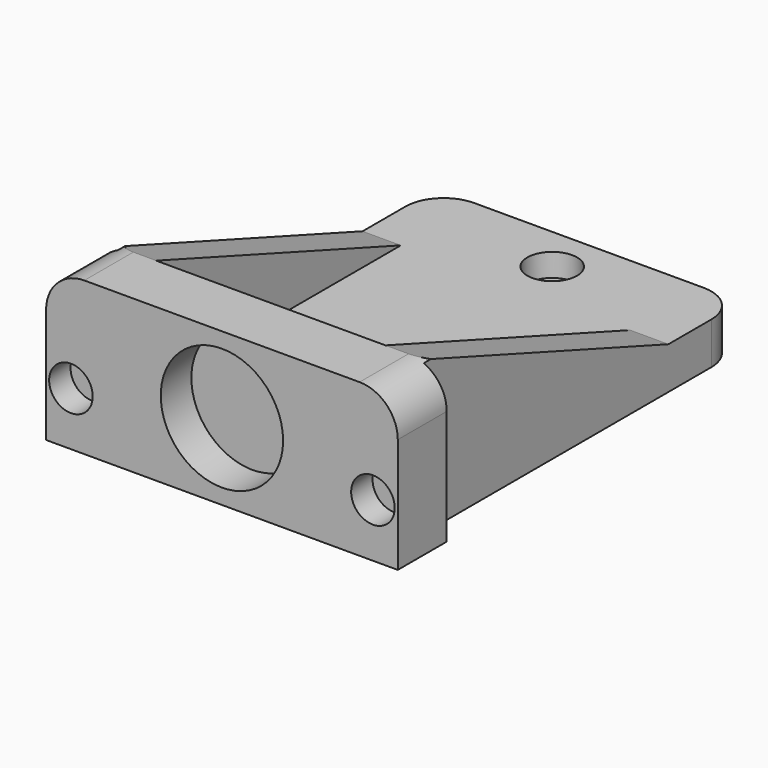
from build123d import *

# Parameters (mm, degrees)
F0_W           = 3
F0_H           = 8
F1_DEPTH       = 20
F0_W_2         = 30
F0_H_2         = 12
F0_H_3         = 40
F0_W_3         = 5
F2_DEPTH       = 5.5
F3_DEPTH       = 20
F5_DEPTH       = 43.001
F7_D           = 3.3
F7_DEPTH       = 13.5002857143
F7_CBORE_D     = 6.5
F7_CBORE_DEPTH = 3
F7_TIP         = 0.9914200214
F8_R           = 8
F9_DEPTH       = 5
F8_R_2         = 2.85
F10_DEPTH      = 3.5
F11_T1_DEPTH   = 30.5
F11_T3_DEPTH   = 33


# Not quite as in the source:
# - a fillet or chamfer that OpenCascade refuses, or shapes differently, is made with other operations: its cross-section is extruded or revolved along the edge and cut away or added


with BuildPart() as f1:
    # F0 (on Top) → F1 (new body)
    with BuildSketch(Plane.XY):
        Polygon((20, -30), (20, -22), (15, -22), (-15, -22), (-20, -22), (-20, -30), align=None)
        with Locations((-21.5, -26)):
            Rectangle(F0_W, F0_H)
        with Locations((21.5, -26)):
            Rectangle(F0_W, F0_H)
    extrude(amount=F1_DEPTH)

    # F0 (on Top) → F2 (join)
    with BuildSketch(Plane.XY):
        with Locations((0, 24)):
            Rectangle(F0_W_2, F0_H_2)
        with Locations((0, -2)):
            Rectangle(F0_W_2, F0_H_3)
        with Locations((-17.5, 24)):
            Rectangle(F0_W_3, F0_H_2)
        with Locations((-17.5, -2)):
            Rectangle(F0_W_3, F0_H_3)
        with Locations((17.5, 24)):
            Rectangle(F0_W_3, F0_H_2)
        with Locations((17.5, -2)):
            Rectangle(F0_W_3, F0_H_3)
    extrude(amount=F2_DEPTH)

    # F0 (on Top) → F3 (join)
    with BuildSketch(Plane.XY):
        with Locations((-17.5, -2)):
            Rectangle(F0_W_3, F0_H_3)
        with Locations((17.5, -2)):
            Rectangle(F0_W_3, F0_H_3)
    extrude(amount=F3_DEPTH)

    # F4 (on face) → F5 (cut, through all)
    with BuildSketch(Plane(origin=(-20, 0, 0), x_dir=(0, -1, 0), z_dir=(-1, 0, 0))):
        Polygon((-18, 20), (-18, 5.5), (22, 20), align=None)
    extrude(amount=-F5_DEPTH, mode=Mode.SUBTRACT)

    # F7
    with Locations(Plane.XY.offset(5.5)):
        with Locations((0, 24), (0, -16)):
            CounterBoreHole(F7_D / 2, F7_CBORE_D / 2, F7_CBORE_DEPTH, depth=F7_DEPTH)
            with Locations((0, 0, -(F7_DEPTH + F7_TIP / 2))):  # 118° drill point
                Cone(0, F7_D / 2, F7_TIP, mode=Mode.SUBTRACT)

    # F8 (on face) → F9 (cut)
    with BuildSketch(Plane.XZ.offset(30)):
        with Locations((0, 10)):
            Circle(F8_R)
    extrude(amount=-F9_DEPTH, mode=Mode.SUBTRACT)

    # F8 (on face) → F10 (cut)
    with BuildSketch(Plane.XZ.offset(30)):
        with Locations((-19.75, 7)):
            Circle(F8_R_2)
        with Locations((19.75, 7)):
            Circle(F8_R_2)
    extrude(amount=-F10_DEPTH, mode=Mode.SUBTRACT)

    # F11: fillet of radius 5 on 4 edges, made by hand

    # F11_s2 → F11_t1 (cut)
    with BuildSketch(Plane.XY.offset(-12.5)):
        with BuildLine():
            ThreePointArc((15, 30), (18.5355339059, 28.5355339059), (20, 25))
            Line((20, 25), (20, 30))
            Line((20, 30), (15, 30))
        make_face()
        with BuildLine():
            ThreePointArc((-20, 25), (-18.5355339059, 28.5355339059), (-15, 30))
            Line((-15, 30), (-20, 30))
            Line((-20, 30), (-20, 25))
        make_face()
    extrude(amount=F11_T1_DEPTH, mode=Mode.SUBTRACT)

    # F11_s4 → F11_t3 (cut)
    with BuildSketch(Plane.XZ.offset(9.5)):
        with BuildLine():
            ThreePointArc((-23, 15), (-21.5355339059, 18.5355339059), (-18, 20))
            Line((-18, 20), (-23, 20))
            Line((-23, 20), (-23, 15))
        make_face()
        with BuildLine():
            ThreePointArc((18, 20), (21.5355339059, 18.5355339059), (23, 15))
            Line((23, 15), (23, 20))
            Line((23, 20), (18, 20))
        make_face()
    extrude(amount=F11_T3_DEPTH, mode=Mode.SUBTRACT)


solid = f1.part
